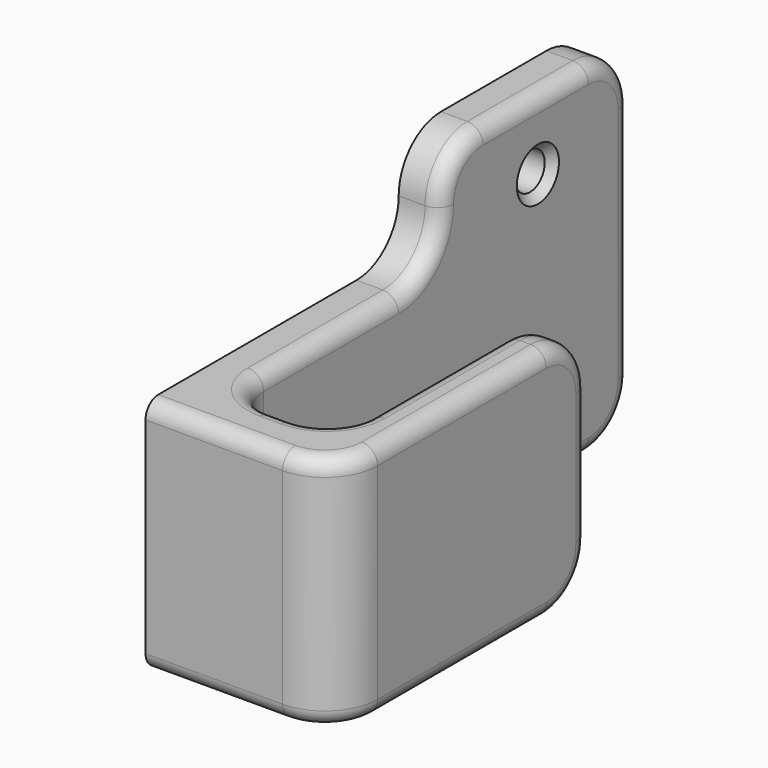
from build123d import *

# Parameters (mm, degrees)
F1_DEPTH       = 45
F2_W           = 45
F2_H           = 65
F3_DEPTH       = 8
F4_R           = 9.99999
F6_R           = 8
F7_R           = 3
F9_D           = 7
F9_CSINK_D     = 10
F9_CSINK_ANGLE = 90


# Not quite as in the source:
# - two fillets or chamfers of one size are made in one step
# - a fillet or chamfer is up to 0.001 mm smaller than in the source, because OpenCascade refuses the exact size


with BuildPart() as f1:
    # F0 (on Top) → F1 (new body)
    with BuildSketch(Plane.XY):
        Polygon((8, 105), (0, 105), (0, 0), (36, 0), (36, 60), (28, 60), (28, 10), (8, 10), align=None)
    extrude(amount=F1_DEPTH)

    # F2 (on Right) → F3 (join, through all)
    with BuildSketch(Plane.YZ):
        with Locations((82.5, 32.5)):
            Rectangle(F2_W, F2_H)
    extrude(amount=F3_DEPTH)

    # F4 (radius 10 in the source; OpenCascade refuses exactly that, so slightly less here)
    f4_edges = [f1.edges().sort_by_distance(p)[0] for p in [
        (4, 60, 45),
        (4, 105, 0),
        (4, 105, 65),
        (4, 60, 65),
        (32, 60, 45),
        (32, 60, 0),
        (36, 0, 22.5),
    ]]
    fillet(f4_edges, radius=F4_R)

    # F6
    f6_edges = [f1.edges().sort_by_distance(p)[0] for p in [
        (8, 10, 22.5),
        (28, 10, 22.5),
    ]]
    fillet(f6_edges, radius=F6_R)

    # F7
    f7_edges = [f1.edges().sort_by_distance(p)[0] for p in [
        (36, 60, 22.5),
        (36, 57.071071, 2.928929),
        (36, 57.071071, 42.071071),
        (36, 30, 0),
        (36, 30, 45),
        (36, 9.99999, 22.5),
        (8, 56.500005, 0),
        (8, 18, 22.5),
        (8, 102.071071, 2.928929),
        (8, 34.000005, 45),
        (8, 105, 32.5),
        (8, 57.071071, 47.928929),
        (8, 102.071071, 62.071071),
        (8, 60, 55),
        (8, 82.5, 65),
        (8, 62.928929, 62.071071),
        (10.343146, 12.343146, 0),
        (18, 10, 0),
        (25.656854, 12.343146, 0),
        (13.000005, 0, 0),
        (28, 34.000005, 0),
        (33.071071, 2.928929, 0),
        (10.343146, 12.343146, 45),
        (18, 10, 45),
        (25.656854, 12.343146, 45),
        (13.000005, 0, 45),
        (28, 34.000005, 45),
        (33.071071, 2.928929, 45),
        (28, 57.071071, 2.928929),
        (28, 60, 22.5),
        (28, 57.071071, 42.071071),
    ]]
    fillet(f7_edges, radius=F7_R)

    # F9 (through all)
    with Locations(Plane.YZ.offset(8)):
        with Locations((83, 51.8898591027), (83, 16.8898591027)):
            CounterSinkHole(F9_D / 2, F9_CSINK_D / 2, counter_sink_angle=F9_CSINK_ANGLE)


solid = f1.part
